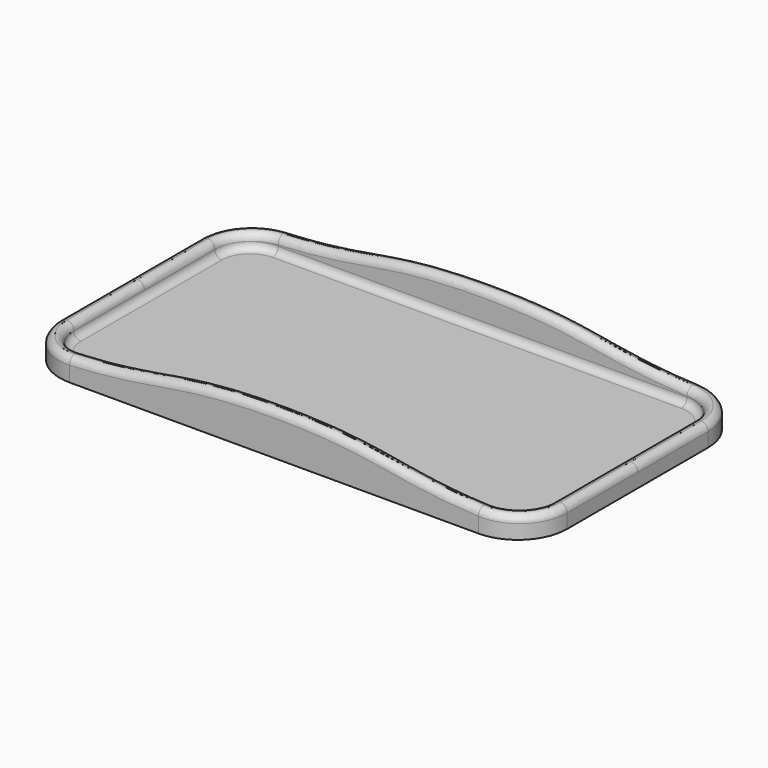
from build123d import *

# Parameters (mm, degrees)
F1_DEPTH = 2
F2_DEPTH = 12
F4_DEPTH = 49.5
F5_R     = 1.9999


# Not quite as in the source:
# - a fillet or chamfer is up to 0.001 mm smaller than in the source, because OpenCascade refuses the exact size


with BuildPart() as f1:
    # F0 (on Top) → F1 (new body)
    with BuildSketch(Plane.XY):
        with BuildLine():
            Line((-58, -35), (58, -35))
            ThreePointArc((58, -35), (65.0710678119, -32.0710678119), (68, -25))
            Line((68, -25), (68, 25))
            ThreePointArc((68, 25), (65.0710678119, 32.0710678119), (58, 35))
            Line((58, 35), (-58, 35))
            ThreePointArc((-58, 35), (-65.0710678119, 32.0710678119), (-68, 25))
            Line((-68, 25), (-68, -25))
            ThreePointArc((-68, -25), (-65.0710678119, -32.0710678119), (-58, -35))
        make_face()
    extrude(amount=F1_DEPTH)

    # F0 (on Top) → F2 (join)
    with BuildSketch(Plane.XY):
        with BuildLine():
            Line((72, -25), (72, 25))
            ThreePointArc((72, 25), (67.8994949366, 34.8994949366), (58, 39))
            Line((58, 39), (-58, 39))
            ThreePointArc((-58, 39), (-67.8994949366, 34.8994949366), (-72, 25))
            Line((-72, 25), (-72, -25))
            ThreePointArc((-72, -25), (-67.8994949366, -34.8994949366), (-58, -39))
            Line((-58, -39), (58, -39))
            ThreePointArc((58, -39), (67.8994949366, -34.8994949366), (72, -25))
        make_face()
        with BuildLine():
            ThreePointArc((68, -25), (65.0710678119, -32.0710678119), (58, -35))
            Line((58, -35), (-58, -35))
            ThreePointArc((-58, -35), (-65.0710678119, -32.0710678119), (-68, -25))
            Line((-68, -25), (-68, 25))
            ThreePointArc((-68, 25), (-65.0710678119, 32.0710678119), (-58, 35))
            Line((-58, 35), (58, 35))
            ThreePointArc((58, 35), (65.0710678119, 32.0710678119), (68, 25))
            Line((68, 25), (68, -25))
        make_face(mode=Mode.SUBTRACT)
    extrude(amount=F2_DEPTH)

    # F3 (on Front) → F4 (intersect, symmetric)
    with BuildSketch(Plane.XZ):
        with BuildLine():
            Line((-72, 0), (72, 0))
            Line((72, 0), (72, 6))
            add(Edge.make_bspline(
                [(72, 6), (33.4486067295, 6), (33.2908295095, 12), (0, 12)],
                knots=[0, 0, 0, 0, 72.2495674728, 72.2495674728, 72.2495674728, 72.2495674728], degree=3))
            add(Edge.make_bspline(
                [(-72, 6), (-33.4486067295, 6), (-33.2908295095, 12), (0, 12)],
                knots=[0, 0, 0, 0, 72.2495674728, 72.2495674728, 72.2495674728, 72.2495674728], degree=3))
            Line((-72, 6), (-72, 0))
        make_face()
    extrude(amount=F4_DEPTH, both=True, mode=Mode.INTERSECT)

    # F5 (radius 2 in the source; OpenCascade refuses exactly that, so slightly less here)
    f5_edges = [f1.edges().sort_by_distance(p)[0] for p in [
        (-68, -25, 4.011282),
        (-65.071068, -32.071068, 2),
        (-58, -35, 4.156731),
        (-65.069672, -32.072463, 6.070191),
        (68.177538, -34.613414, 6.020562),
        (72, -12.5, 6),
        (29.762473, -39, 9.705642),
        (29.762473, -35, 9.705642),
        (65.256612, -31.880522, 6.066302),
        (68, -12.5, 6.022564),
        (68, 12.5, 6.022564),
        (68, 0, 2),
        (0, -35, 2),
        (65.071068, -32.071068, 2),
        (65.071068, 32.071068, 2),
        (0, 35, 2),
        (-65.071068, 32.071068, 2),
        (-68, 0, 2),
        (-68, 12.5, 6.022564),
        (-68, -12.5, 6.022564),
        (-29.762473, 35, 9.705642),
        (-65.256612, 31.880522, 6.066302),
        (-72, 12.5, 6),
        (-68.177538, 34.613414, 6.020562),
        (-29.762473, 39, 9.705642),
        (29.762473, 35, 9.705642),
        (65.256612, 31.880522, 6.066302),
        (-29.762473, -35, 9.705642),
        (-72, -12.5, 6),
        (-68.177538, -34.613414, 6.020562),
        (-29.762473, -39, 9.705642),
        (72, 12.5, 6),
        (68.177538, 34.613414, 6.020562),
        (29.762473, 39, 9.705642),
    ]]
    fillet(f5_edges, radius=F5_R)


solid = f1.part
